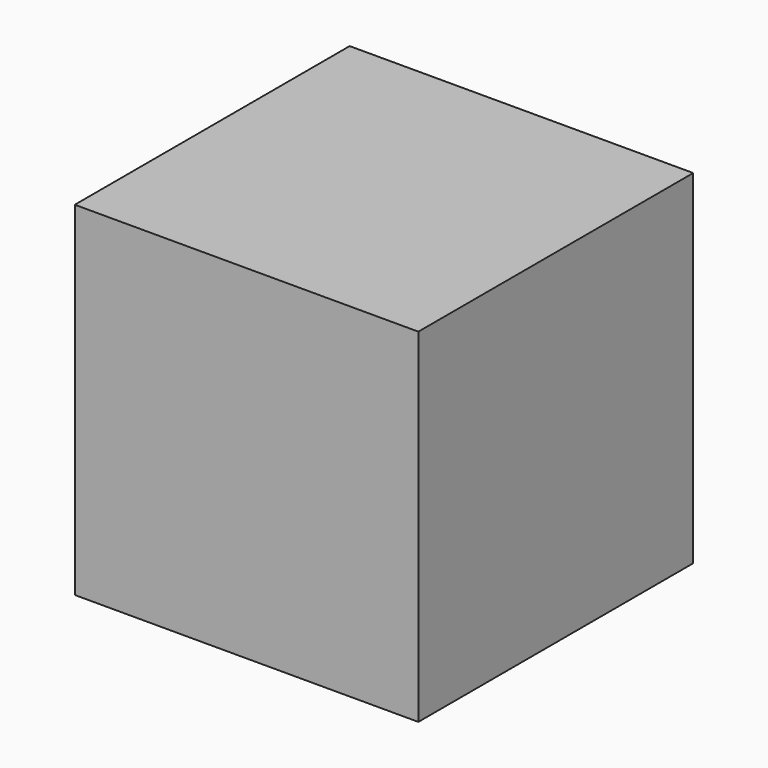
from build123d import *

# Parameters (mm, degrees)
F1_W     = 101.6
F1_H     = 101.6
F2_DEPTH = 50.8


# Not quite as in the source:
# - a variable given as a bare number and used for a length is read in inches; the dataset says mm whatever the document's units were


with BuildPart() as f2:
    # F1 (on Front) → F2 (new body, symmetric)
    with BuildSketch(Plane.XZ):
        Rectangle(F1_W, F1_H)
    extrude(amount=F2_DEPTH, both=True)


solid = f2.part
